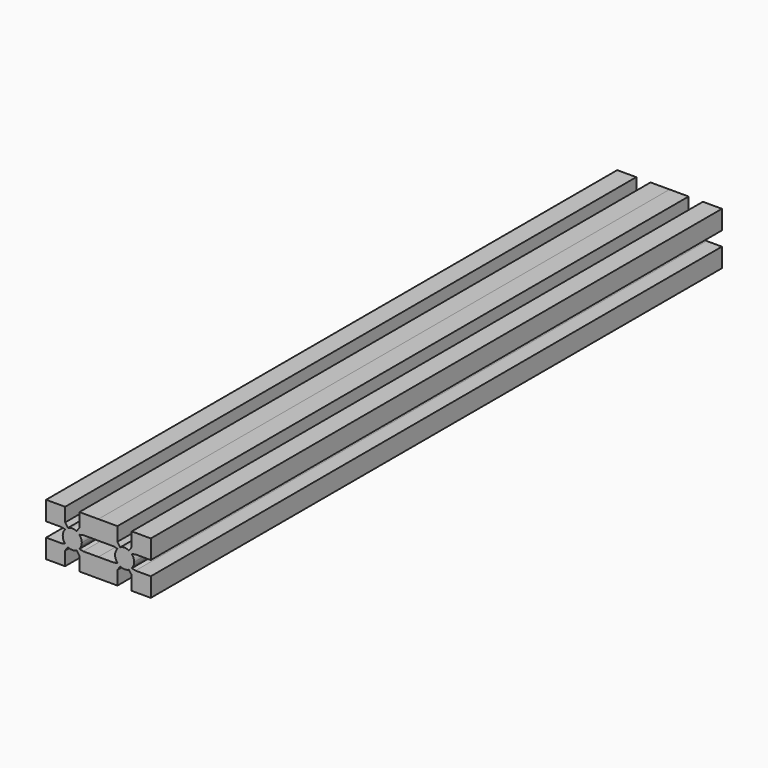
from build123d import *

# Parameters (mm, degrees)
F1_DEPTH = 600


# Not quite as in the source:
# - ends of sketch curves that miss each other by under 0.0002 mm in the source are joined


with BuildPart() as f1:
    # F0 (on Front) → F1 (new body)
    with BuildSketch(Plane.XZ):
        with BuildLine():
            Line((25.9504089346, 7.0230446355), (41.9504089346, 7.0230446355))
            Line((41.9504089346, 7.0230446355), (41.9504085783, 23.0230446355))
            Line((41.9504085783, 23.0230446355), (29.0776360335, 23.0230446355))
            Line((29.0776360335, 23.0230446355), (25.9629066643, 23.7457469321))
            ThreePointArc((25.9629066643, 23.7457469321), (24.8732485493, 22.7170435153), (23.6108614125, 21.9096004868))
            Line((23.6108614125, 21.9096004868), (25.9504089346, 18.5945479171))
            Line((25.9504089346, 18.5945479171), (25.9504089346, 7.0230446355))
        make_face()
        with BuildLine():
            ThreePointArc((16.2899564567, 21.9096004868), (19.9504089346, 21.0230446355), (23.6108614125, 21.9096004868))
            ThreePointArc((23.6108614125, 21.9096004868), (24.8732485493, 22.7170435153), (25.9629066643, 23.7457469321))
            ThreePointArc((25.9629066643, 23.7457469321), (27.4370631218, 26.2034685892), (27.9504089346, 29.0230446355))
            ThreePointArc((27.9504089346, 29.0230446355), (27.4370631218, 31.8426206818), (25.9629066643, 34.3003423389))
            ThreePointArc((25.9629066643, 34.3003423389), (24.8732485493, 35.3290457557), (23.6108614125, 36.1364887842))
            ThreePointArc((23.6108614125, 36.1364887842), (19.9504089346, 37.0230446355), (16.2899564567, 36.1364887842))
            ThreePointArc((16.2899564567, 36.1364887842), (15.0275693199, 35.3290457557), (13.9379112049, 34.3003423389))
            ThreePointArc((13.9379112049, 34.3003423389), (11.9504089346, 29.0230446355), (13.9379112049, 23.7457469321))
            ThreePointArc((13.9379112049, 23.7457469321), (15.0275693199, 22.7170435153), (16.2899564567, 21.9096004868))
        make_face()
        with BuildLine():
            Line((13.9504089346, 18.5945479171), (16.2899564567, 21.9096004868))
            ThreePointArc((16.2899564567, 21.9096004868), (15.0275693199, 22.7170435153), (13.9379112049, 23.7457469321))
            Line((13.9379112049, 23.7457469321), (10.8231818357, 23.0230446355))
            Line((10.8231818357, 23.0230446355), (-2.0495907091, 23.0230446355))
            Line((-2.0495907091, 23.0230446355), (-2.0495910654, 7.0230446355))
            Line((-2.0495910654, 7.0230446355), (13.9504089346, 7.0230446355))
            Line((13.9504089346, 7.0230446355), (13.9504089346, 18.5945479171))
        make_face()
        with BuildLine():
            ThreePointArc((23.6108614125, 36.1364887842), (24.8732485493, 35.3290457557), (25.9629066643, 34.3003423389))
            Line((25.9629066643, 34.3003423389), (29.0776360335, 35.0230446355))
            Line((29.0776360335, 35.0230446355), (41.9504085783, 35.0230446355))
            Line((41.9504085783, 35.0230446355), (41.9504089346, 51.0230446355))
            Line((41.9504089346, 51.0230446355), (25.9504089346, 51.0230446355))
            Line((25.9504089346, 51.0230446355), (25.9504089346, 39.4515413539))
            Line((25.9504089346, 39.4515413539), (23.6108614125, 36.1364887842))
        make_face()
        with BuildLine():
            Line((10.8231818357, 35.0230446355), (13.9379112049, 34.3003423389))
            ThreePointArc((13.9379112049, 34.3003423389), (15.0275693199, 35.3290457557), (16.2899564567, 36.1364887842))
            Line((16.2899564567, 36.1364887842), (13.9504089346, 39.4515413539))
            Line((13.9504089346, 39.4515413539), (13.9504089346, 51.0230446355))
            Line((13.9504089346, 51.0230446355), (-2.0495910654, 51.0230446355))
            Line((-2.0495910654, 51.0230446355), (-2.0495907091, 35.0230446355))
            Line((-2.0495907091, 35.0230446355), (10.8231818357, 35.0230446355))
        make_face()
        with BuildLine():
            Line((-2.0495910654, 7.0230446355), (-2.0495907091, 23.0230446355))
            Line((-2.0495907091, 23.0230446355), (-14.9223627195, 23.0230440622))
            Line((-14.9223627195, 23.0230440622), (-18.0370921209, 23.7457462201))
            ThreePointArc((-18.0370921209, 23.7457462201), (-19.1267501901, 22.7170427548), (-20.389137291, 21.90959967))
            Line((-20.389137291, 21.90959967), (-18.0495896212, 18.5945472045))
            Line((-18.0495896212, 18.5945472045), (-18.0495891058, 7.0230439229))
            Line((-18.0495891058, 7.0230439229), (-2.0495910654, 7.0230446355))
        make_face()
        with BuildLine():
            Line((-14.9223632539, 35.0230440622), (-2.0495907091, 35.0230446355))
            Line((-2.0495907091, 35.0230446355), (-2.0495910654, 51.0230446355))
            Line((-2.0495910654, 51.0230446355), (-18.0495910654, 51.0230439229))
            Line((-18.0495910654, 51.0230439229), (-18.0495905501, 39.4515406413))
            Line((-18.0495905501, 39.4515406413), (-20.3891379246, 36.1364879675))
            ThreePointArc((-20.3891379246, 36.1364879675), (-19.1267507518, 35.3290449952), (-18.0370925909, 34.3003416269))
            Line((-18.0370925909, 34.3003416269), (-14.9223632539, 35.0230440622))
        make_face()
        with BuildLine():
            ThreePointArc((-20.389137291, 21.90959967), (-19.1267501901, 22.7170427548), (-18.0370921209, 23.7457462201))
            ThreePointArc((-18.0370921209, 23.7457462201), (-16.5629358356, 26.2034677761), (-16.0495900856, 29.0230436557))
            ThreePointArc((-16.0495900856, 29.0230436557), (-16.5629359612, 31.8426198688), (-18.0370925909, 34.3003416269))
            ThreePointArc((-18.0370925909, 34.3003416269), (-19.1267507518, 35.3290449952), (-20.3891379246, 36.1364879675))
            ThreePointArc((-20.3891379246, 36.1364879675), (-24.0495904419, 37.0230436557), (-27.7100428803, 36.1364876414))
            ThreePointArc((-27.7100428803, 36.1364876414), (-28.9724299811, 35.3290445567), (-30.0620880504, 34.3003410913))
            ThreePointArc((-30.0620880504, 34.3003410913), (-32.0495900856, 29.0230432994), (-30.0620875803, 23.7457456846))
            ThreePointArc((-30.0620875803, 23.7457456846), (-28.9724294195, 22.7170423163), (-27.7100422467, 21.909599344))
            ThreePointArc((-27.7100422467, 21.909599344), (-24.0495897293, 21.0230436557), (-20.389137291, 21.90959967))
        make_face()
        with BuildLine():
            Line((-30.0495896212, 18.5945466701), (-27.7100422467, 21.909599344))
            ThreePointArc((-27.7100422467, 21.909599344), (-28.9724294195, 22.7170423163), (-30.0620875803, 23.7457456846))
            Line((-30.0620875803, 23.7457456846), (-33.1768169173, 23.0230432492))
            Line((-33.1768169173, 23.0230432492), (-46.0495894621, 23.0230426759))
            Line((-46.0495894621, 23.0230426759), (-46.0495891058, 7.0230426759))
            Line((-46.0495891058, 7.0230426759), (-30.0495891058, 7.0230433885))
            Line((-30.0495891058, 7.0230433885), (-30.0495896212, 18.5945466701))
        make_face()
        with BuildLine():
            ThreePointArc((-30.0620880504, 34.3003410913), (-28.9724299811, 35.3290445567), (-27.7100428803, 36.1364876414))
            Line((-27.7100428803, 36.1364876414), (-30.0495905501, 39.4515401069))
            Line((-30.0495905501, 39.4515401069), (-30.0495910654, 51.0230433885))
            Line((-30.0495910654, 51.0230433885), (-46.0495910654, 51.0230426759))
            Line((-46.0495910654, 51.0230426759), (-46.0495899966, 35.0230426759))
            Line((-46.0495899966, 35.0230426759), (-33.1768174518, 35.0230432492))
            Line((-33.1768174518, 35.0230432492), (-30.0620880504, 34.3003410913))
        make_face()
    extrude(amount=F1_DEPTH)


solid = f1.part
